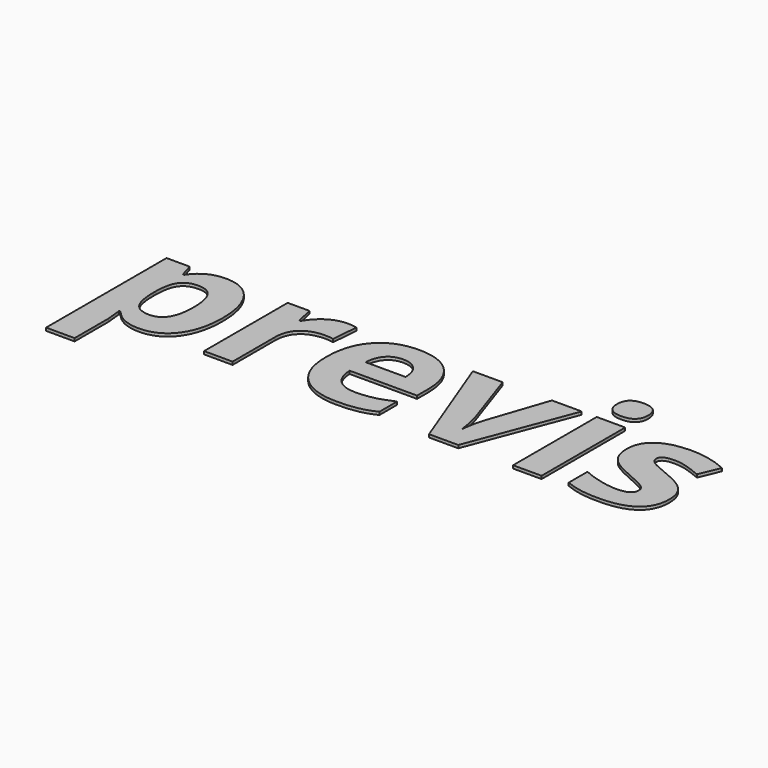
from build123d import *

# Parameters (mm, degrees)
F0_TEXT_SIZE = 16.2568583621
F1_DEPTH     = 0.25


# Not quite as in the source:
# - Text() gives the source's letters only with a copy of the font that has no kerning and outlines rounded to 1/6400 em; it was checked with that copy


with BuildPart() as f1:
    # F0 (on Top) → F1 (new body)
    with BuildSketch(Plane.XY):
        with Locations((-25, -5.0077827585)):
            Text('previs', F0_TEXT_SIZE, font='Open Sans', font_style=FontStyle.BOLD, text_align=(TextAlign.LEFT, TextAlign.BOTTOM))
    extrude(amount=F1_DEPTH)


solid = f1.part
